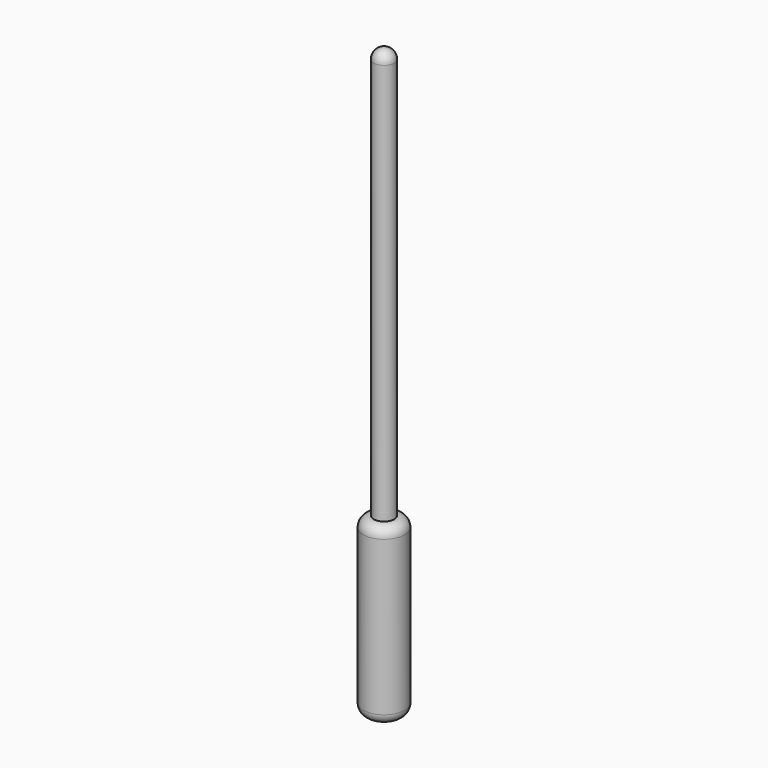
from build123d import *

# Parameters (mm, degrees)
F0_R     = 5
F1_DEPTH = 200
F2_R     = 10
F2_R_2   = 5
F3_DEPTH = 85
F4_R     = 4.99999
F5_R     = 5


# Not quite as in the source:
# - a fillet or chamfer is up to 0.001 mm smaller than in the source, because OpenCascade refuses the exact size


with BuildPart() as f1:
    # F0 (on Top) → F1 (new body)
    with BuildSketch(Plane.XY):
        Circle(F0_R)
    extrude(amount=F1_DEPTH)

    # F2 (on face) → F3 (join)
    with BuildSketch(Plane(origin=(0, 0, 0), x_dir=(1, 0, 0), z_dir=(0, 0, -1))):
        Circle(F2_R)
        Circle(F2_R_2, mode=Mode.SUBTRACT)
        Circle(F2_R_2)
    extrude(amount=F3_DEPTH)

    # F4 (radius 5 in the source; OpenCascade refuses exactly that, so slightly less here)
    f4_edges = [f1.edges().sort_by_distance(p)[0] for p in [
        (-10, 0, 0),
        (-10, 0, -85),
    ]]
    fillet(f4_edges, radius=F4_R)

    # F5
    f5_edges = [f1.edges().sort_by_distance(p)[0] for p in [
        (-5, 0, 200),
    ]]
    fillet(f5_edges, radius=F5_R)


solid = f1.part
